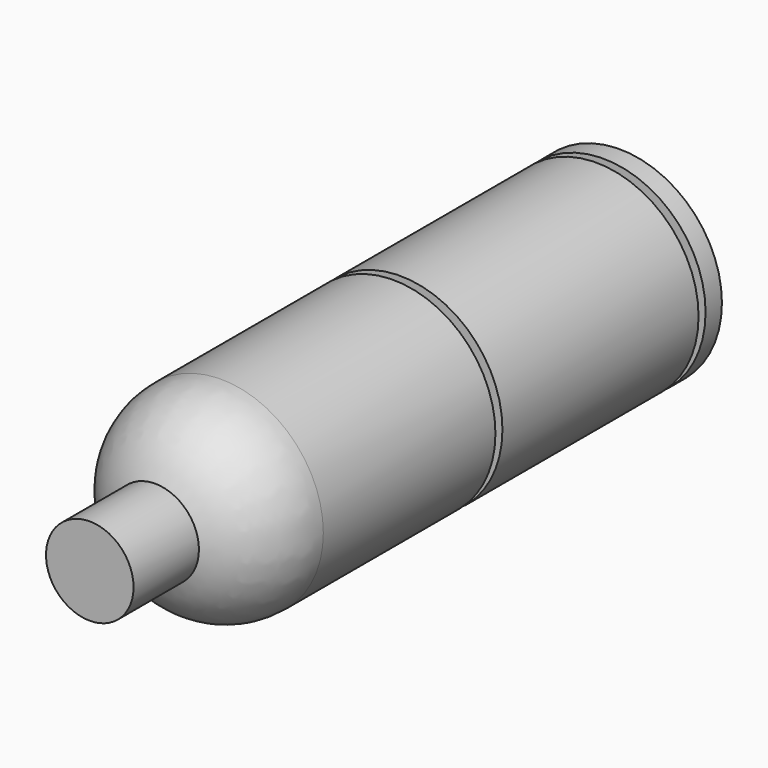
from build123d import *

# Parameters (mm, degrees)
F0_R     = 35
F1_DEPTH = 230
F3_R     = 40.5
F3_R_2   = 30.5
F4_DEPTH = 3
F6_R     = 36.6776
F6_R_2   = 30.5
F7_DEPTH = 3
F8_R     = 38.3794
F8_R_2   = 15
F9_DEPTH = 28


# Not quite as in the source:
# - a fillet or chamfer that OpenCascade refuses, or shapes differently, is made with other operations: its cross-section is extruded or revolved along the edge and cut away or added


with BuildPart() as f1:
    # F0 (on Front) → F1 (new body)
    with BuildSketch(Plane.XZ):
        Circle(F0_R)
    extrude(amount=F1_DEPTH)

    # F3 (on offset) + F0 (on Front) → F4 (cut)
    with BuildSketch(Plane(origin=(0, -10, 0), x_dir=(-1, 0, 0), z_dir=(0, 1, 0))):
        Circle(F3_R)
        Circle(F3_R_2, mode=Mode.SUBTRACT)
    with BuildSketch(Plane.XZ):
        Circle(F0_R)
    extrude(amount=-F4_DEPTH, dir=(0, 1, 0), mode=Mode.SUBTRACT)

    # F6 (on offset) → F7 (cut)
    with BuildSketch(Plane(origin=(0, -97, 0), x_dir=(-1, 0, 0), z_dir=(0, 1, 0))):
        Circle(F6_R)
        Circle(F6_R_2, mode=Mode.SUBTRACT)
    extrude(amount=-F7_DEPTH, mode=Mode.SUBTRACT)

    # F8 (on face) → F9 (cut)
    with BuildSketch(Plane.XZ.offset(230)):
        Circle(F8_R)
        Circle(F8_R_2, mode=Mode.SUBTRACT)
    extrude(amount=-F9_DEPTH, mode=Mode.SUBTRACT)

    # F10: fillet of radius 30 on 1 edges, made by hand

    # F10_s1 → F10_t2 (revolve, cut)
    with BuildSketch(Plane.XY):
        with BuildLine():
            ThreePointArc((35, -173.7157287525), (29.4948974278, -191.0362368282), (15, -202))
            Line((15, -202), (35, -202))
            Line((35, -202), (35, -173.7157287525))
        make_face()
    revolve(axis=Axis((0, -202, 0), (0, 1, 0)), mode=Mode.SUBTRACT)


solid = f1.part
